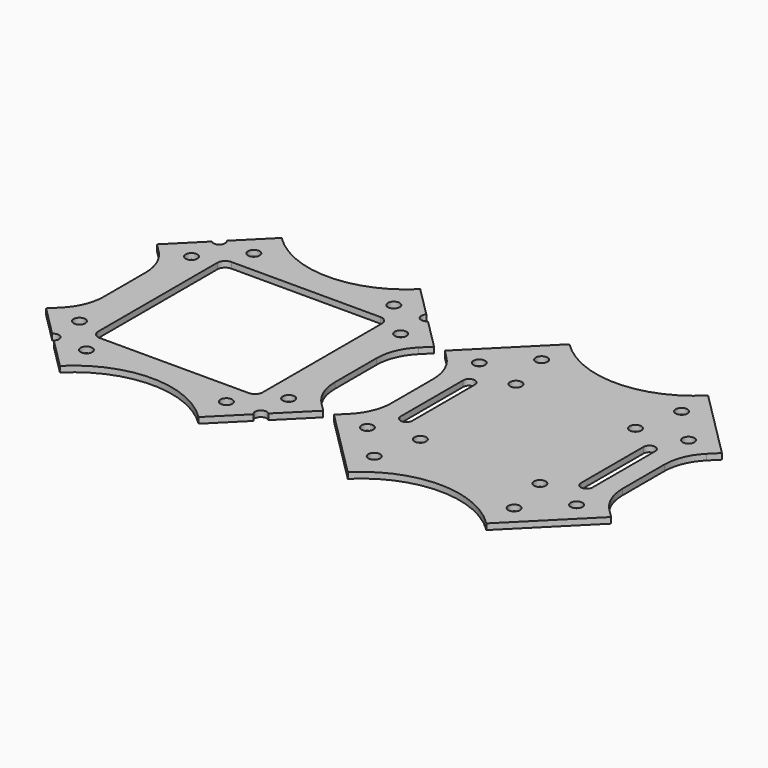
from build123d import *

# Parameters (mm, degrees)
F0_R     = 1.5
F1_DEPTH = 1.5


# Not quite as in the source:
# - ends of sketch curves that miss each other by under 0.0002 mm in the source are joined


with BuildPart() as f1:
    # F0 (on Top) → F1 (new body)
    with BuildSketch(Plane.XY):
        with BuildLine():
            Line((-66.21884, 6.64466), (-66.21884, -1e-06))
            Line((-66.21884, -1e-06), (-66.21884, -6.644662))
            ThreePointArc((-66.21884, -6.644662), (-67.1703457083, -11.4282045779), (-69.8800047352, -15.4834962648))
            Line((-69.8800047352, -15.4834962648), (-72.074179, -17.67767))
            Line((-72.074179, -17.67767), (-64.296005, -25.455845))
            ThreePointArc((-64.296005, -25.455845), (-62.1746850782, -25.4558445782), (-62.1746843282, -27.5771646718))
            Line((-62.1746843282, -27.5771646718), (-54.39651, -35.35534))
            ThreePointArc((-54.39651, -35.35534), (-36.7188403536, -28.033009), (-19.0411704703, -35.3553394703))
            Line((-19.0411704703, -35.3553394703), (-11.262996, -27.577165))
            ThreePointArc((-11.262996, -27.577165), (-11.2629961718, -25.4558448282), (-9.1416758282, -25.4558448282))
            Line((-9.1416758282, -25.4558448282), (-1.363501, -17.67767))
            Line((-1.363501, -17.67767), (-3.557675, -15.483496))
            ThreePointArc((-3.557675, -15.483496), (-6.2673342917, -11.4282045779), (-7.21884, -6.644662))
            Line((-7.21884, -6.644662), (-7.21884, -1e-06))
            Line((-7.21884, -1e-06), (-7.21884, 6.64466))
            ThreePointArc((-7.21884, 6.64466), (-6.2673341564, 11.4282029046), (-3.5576747648, 15.4834947648))
            Line((-3.5576747648, 15.4834947648), (-1.363501, 17.677669))
            Line((-1.363501, 17.677669), (-9.141676, 25.455843))
            ThreePointArc((-9.141676, 25.455843), (-11.2629964218, 25.4558440782), (-11.2629961718, 27.5771641718))
            Line((-11.2629961718, 27.5771641718), (-19.041171, 35.355338))
            ThreePointArc((-19.041171, 35.355338), (-36.7188403536, 28.033008), (-54.3965095297, 35.3553384703))
            Line((-54.3965095297, 35.3553384703), (-62.174684, 27.577164))
            ThreePointArc((-62.174684, 27.577164), (-62.1746848282, 25.4558438282), (-64.2960046718, 25.4558433282))
            Line((-64.2960046718, 25.4558433282), (-72.074179, 17.677669))
            Line((-72.074179, 17.677669), (-69.880005, 15.483495))
            ThreePointArc((-69.880005, 15.483495), (-67.1703458436, 11.4282029046), (-66.21884, 6.64466))
        make_face()
        with Locations((-54.573286, -26.693282)):
            Circle(F0_R, mode=Mode.SUBTRACT)
        with Locations((-63.412121, -17.854447)):
            Circle(F0_R, mode=Mode.SUBTRACT)
        with Locations((-18.864394, -26.693282)):
            Circle(F0_R, mode=Mode.SUBTRACT)
        with Locations((-10.025559, -17.854447)):
            Circle(F0_R, mode=Mode.SUBTRACT)
        with BuildLine():
            ThreePointArc((-57.71884, 18.999999), (-57.1330535624, 20.4142125624), (-55.71884, 20.999999))
            Line((-55.71884, 20.999999), (-17.71884, 20.999999))
            ThreePointArc((-17.71884, 20.999999), (-16.3046264376, 20.4142125624), (-15.71884, 18.999999))
            Line((-15.71884, 18.999999), (-15.71884, -19.000001))
            ThreePointArc((-15.71884, -19.000001), (-16.3046264376, -20.4142145624), (-17.71884, -21.000001))
            Line((-17.71884, -21.000001), (-55.71884, -21.000001))
            ThreePointArc((-55.71884, -21.000001), (-57.1330535624, -20.4142145624), (-57.71884, -19.000001))
            Line((-57.71884, -19.000001), (-57.71884, 18.999999))
        make_face(mode=Mode.SUBTRACT)
        with Locations((-63.412121, 17.854446)):
            Circle(F0_R, mode=Mode.SUBTRACT)
        with Locations((-54.573286, 26.69328)):
            Circle(F0_R, mode=Mode.SUBTRACT)
        with Locations((-10.025559, 17.854446)):
            Circle(F0_R, mode=Mode.SUBTRACT)
        with Locations((-18.864394, 26.69328)):
            Circle(F0_R, mode=Mode.SUBTRACT)
    extrude(amount=F1_DEPTH)


with BuildPart() as f1b:
    # F0 (on Top) → F1, piece 2 (new body)
    with BuildSketch(Plane.XY):
        with BuildLine():
            Line((7.218841, 6.644661), (7.218841, 0))
            Line((7.218841, 0), (7.218841, -6.64466))
            ThreePointArc((7.218841, -6.64466), (6.2673351564, -11.4282029046), (3.5576757648, -15.4834947648))
            Line((3.5576757648, -15.4834947648), (1.363502, -17.677669))
            Line((1.363502, -17.677669), (19.041171, -35.355339))
            ThreePointArc((19.041171, -35.355339), (36.7188406464, -28.033008), (54.3965105297, -35.3553384703))
            Line((54.3965105297, -35.3553384703), (72.07418, -17.677669))
            Line((72.07418, -17.677669), (69.880006, -15.483495))
            ThreePointArc((69.880006, -15.483495), (67.1703468436, -11.4282029046), (66.218841, -6.64466))
            Line((66.218841, -6.64466), (66.218841, 0))
            Line((66.218841, 0), (66.218841, 6.644661))
            ThreePointArc((66.218841, 6.644661), (67.1703468436, 11.4282039046), (69.8800062352, 15.4834957648))
            Line((69.8800062352, 15.4834957648), (72.07418, 17.67767))
            Line((72.07418, 17.67767), (54.39651, 35.35534))
            ThreePointArc((54.39651, 35.35534), (36.7188406464, 28.033009), (19.0411709703, 35.3553399703))
            Line((19.0411709703, 35.3553399703), (1.363502, 17.67767))
            Line((1.363502, 17.67767), (3.557676, 15.483496))
            ThreePointArc((3.557676, 15.483496), (6.2673351564, 11.4282039046), (7.218841, 6.644661))
        make_face()
        with Locations((18.864395, -26.69328)):
            Circle(F0_R, mode=Mode.SUBTRACT)
        with Locations((10.02556, -17.854446)):
            Circle(F0_R, mode=Mode.SUBTRACT)
        with Locations((54.573287, -26.69328)):
            Circle(F0_R, mode=Mode.SUBTRACT)
        with Locations((63.412122, -17.854446)):
            Circle(F0_R, mode=Mode.SUBTRACT)
        with Locations((21.468841, -15.25)):
            Circle(F0_R, mode=Mode.SUBTRACT)
        with Locations((51.968841, -15.25)):
            Circle(F0_R, mode=Mode.SUBTRACT)
        with BuildLine():
            ThreePointArc((15.218841, -10), (13.718841, -11.5), (12.218841, -10))
            Line((12.218841, -10), (12.218841, 0))
            Line((12.218841, 0), (12.218841, 10))
            ThreePointArc((12.218841, 10), (13.718841, 11.5), (15.218841, 10))
            Line((15.218841, 10), (15.218841, 0))
            Line((15.218841, 0), (15.218841, -10))
        make_face(mode=Mode.SUBTRACT)
        with Locations((21.468841, 15.25)):
            Circle(F0_R, mode=Mode.SUBTRACT)
        with BuildLine():
            ThreePointArc((61.218841, -10), (59.718841, -11.5), (58.218841, -10))
            Line((58.218841, -10), (58.218841, 0))
            Line((58.218841, 0), (58.218841, 10))
            ThreePointArc((58.218841, 10), (59.718841, 11.5), (61.218841, 10))
            Line((61.218841, 10), (61.218841, 0))
            Line((61.218841, 0), (61.218841, -10))
        make_face(mode=Mode.SUBTRACT)
        with Locations((51.968841, 15.25)):
            Circle(F0_R, mode=Mode.SUBTRACT)
        with Locations((10.02556, 17.854447)):
            Circle(F0_R, mode=Mode.SUBTRACT)
        with Locations((18.864395, 26.693281)):
            Circle(F0_R, mode=Mode.SUBTRACT)
        with Locations((63.412122, 17.854447)):
            Circle(F0_R, mode=Mode.SUBTRACT)
        with Locations((54.573287, 26.693281)):
            Circle(F0_R, mode=Mode.SUBTRACT)
    extrude(amount=F1_DEPTH)


solid = Compound([f1.part, f1b.part])
